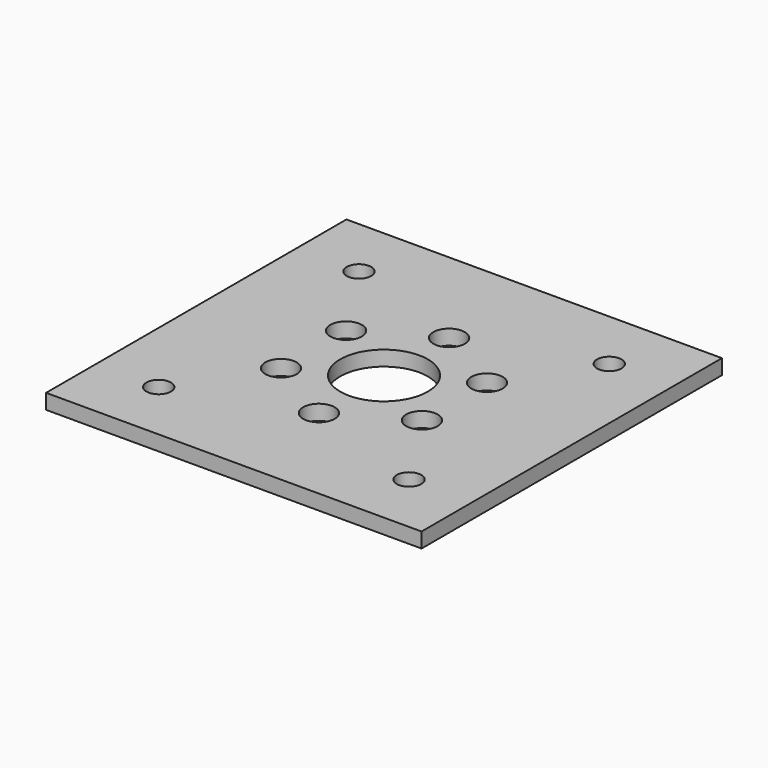
from build123d import *

# Parameters (mm, degrees)
F0_R            = 41.5
F1_DEPTH        = 6
F2_W            = 150
F2_H            = 150
F3_DEPTH        = 6
F5_R            = 17.5
F6_DEPTH        = 6.001
F7_D            = 12.6
F7_COPIES_COUNT = 6
F9_D            = 9.8044


# Not quite as in the source:
# - a pattern or mirror of a feature is missing from the dataset's text; its kind, count and spacing are read off the source's solid


with BuildPart() as f1:
    # F0 (on Top) → F1 (new body)
    with BuildSketch(Plane.XY):
        Circle(F0_R)
    extrude(amount=F1_DEPTH)

    # F2 (on Top) → F3 (join)
    with BuildSketch(Plane.XY):
        Rectangle(F2_W, F2_H)
    extrude(amount=F3_DEPTH)

    # F5 (on face) → F6 (cut, through all)
    with BuildSketch(Plane.XY.offset(6)):
        Circle(F5_R)
    extrude(amount=-F6_DEPTH, mode=Mode.SUBTRACT)

    # F7 (through all)
    with Locations(Plane.XY.offset(6)):
        with Locations((0, 32.5)):
            f7 = Hole(F7_D / 2)

    # F7_copies: F7 ×6 about axis
    f7_copies_axis = Axis((0, 0, 0), (0, 0, 1))
    for i in range(1, F7_COPIES_COUNT):
        add(f7.rotate(f7_copies_axis, i * 360 / F7_COPIES_COUNT), mode=Mode.SUBTRACT)

    # F9 (through all)
    with Locations(Plane.XY.offset(6)):
        with Locations((-50, 50), (50, 50), (50, -50), (-50, -50)):
            Hole(F9_D / 2)


solid = f1.part
